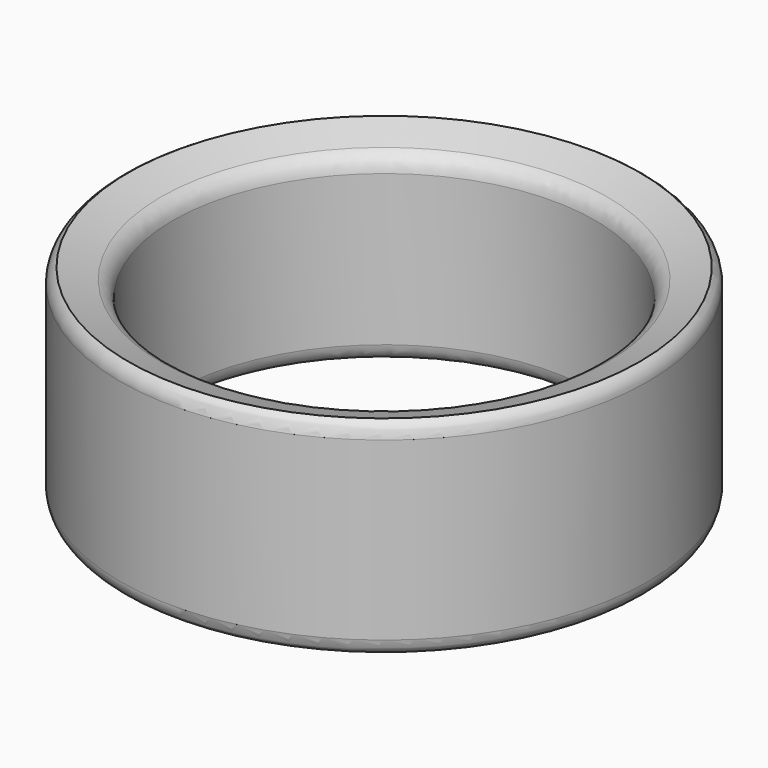
from build123d import *

# Parameters (mm, degrees)
F2_R     = 10
F2_R_2   = 8
F3_DEPTH = 8
F4_R     = 0.6666666667
F6_R     = 0.6666666667


# Not quite as in the source:
# - a fillet or chamfer that OpenCascade refuses, or shapes differently, is made with other operations: its cross-section is extruded or revolved along the edge and cut away or added


with BuildPart() as f3:
    # F2 (on Top) → F3 (new body)
    with BuildSketch(Plane.XY):
        Circle(F2_R)
        Circle(F2_R_2, mode=Mode.SUBTRACT)
    extrude(amount=F3_DEPTH)

    # F4
    f4_edges = [f3.edges().sort_by_distance(p)[0] for p in [
        (-10, 0, 8),
        (-10, 0, 0),
    ]]
    fillet(f4_edges, radius=F4_R)

    # F5: chamfer of 2 x 0.6666666667 on 2 edges, made by hand

    # F5_s1 → F5_t2 (revolve, cut)
    with BuildSketch(Plane.XZ):
        Polygon((10, 0), (8, 0.6666666667), (8, 0), align=None)
    revolve(axis=Axis((0, 0, 0), (0, 0, 1)), mode=Mode.SUBTRACT)

    # F5_s3 → F5_t4 (revolve, cut)
    with BuildSketch(Plane.XZ):
        Polygon((10, 8), (8, 7.3333333333), (8, 8), align=None)
    revolve(axis=Axis((0, 0, 8), (0, 0, 1)), mode=Mode.SUBTRACT)

    # F6
    f6_edges = [f3.edges().sort_by_distance(p)[0] for p in [
        (-8, 0, 7.333333),
        (-8, 0, 0.666667),
    ]]
    fillet(f6_edges, radius=F6_R)


solid = f3.part
